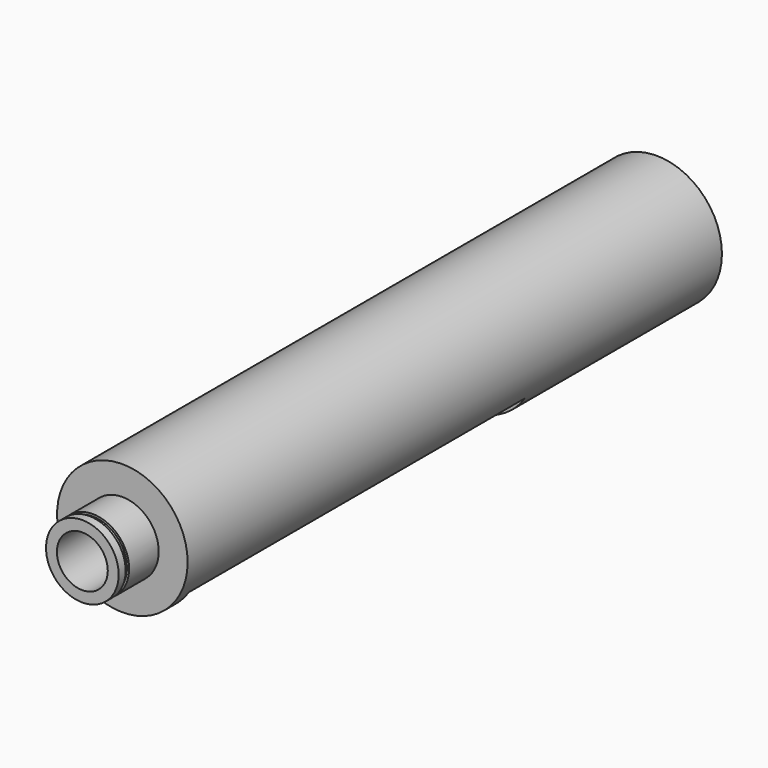
from build123d import *

# Parameters (mm, degrees)
F0_R      = 8.35
F0_R_2    = 5.85
F1_DEPTH  = 15
F2_START  = -11.5
F0_R_3    = 15
F0_R_4    = 12.5
F2_DEPTH  = 3.5
F3_START  = -15
F3_DEPTH  = 150
F4_R      = 15
F4_R_2    = 12.5
F5_DEPTH  = 5
F7_START  = -5
F7_DEPTH  = 51
F8_DEPTH  = 61
F6_W      = 2.95
F6_H      = 4.6
F9_DEPTH  = 15.5
F12_DEPTH = 25
F14_DEPTH = 18.0629715323
F15_DEPTH = 3
F17_START = -2
F16_R     = 8.35
F16_R_2   = 7.85
F17_DEPTH = 1


with BuildPart() as f1:
    # F0 (on Front) → F1 (new body)
    with BuildSketch(Plane.XZ):
        with Locations((-30.6610018015, 20.1133023947)):
            Circle(F0_R)
        with Locations((-30.6610018015, 20.1133023947)):
            Circle(F0_R_2, mode=Mode.SUBTRACT)
    extrude(amount=-F1_DEPTH)

    # F0 (on Front) → F2 (join)
    with BuildSketch(Plane.XZ.offset(F2_START)):
        with Locations((-30.6610018015, 20.1133023947)):
            Circle(F0_R_3)
        with Locations((-30.6610018015, 20.1133023947)):
            Circle(F0_R_4, mode=Mode.SUBTRACT)
        with Locations((-30.6610018015, 20.1133023947)):
            Circle(F0_R_4)
        with Locations((-30.6610018015, 20.1133023947)):
            Circle(F0_R, mode=Mode.SUBTRACT)
    extrude(amount=-F2_DEPTH)

    # F0 (on Front) → F3 (join)
    with BuildSketch(Plane.XZ.offset(F3_START)):
        with Locations((-30.6610018015, 20.1133023947)):
            Circle(F0_R_3)
        with Locations((-30.6610018015, 20.1133023947)):
            Circle(F0_R_4, mode=Mode.SUBTRACT)
    extrude(amount=-F3_DEPTH)

    # F4 (on face) → F5 (join)
    with BuildSketch(Plane(origin=(0, 165, 0), x_dir=(-1, 0, 0), z_dir=(0, 1, 0))):
        with Locations((30.6610018015, 20.1133023947)):
            Circle(F4_R)
        with Locations((30.6610018015, 20.1133023947)):
            Circle(F4_R_2, mode=Mode.SUBTRACT)
        with Locations((30.6610018015, 20.1133023947)):
            Circle(F4_R_2)
    extrude(amount=-F5_DEPTH)

    # F6 (on face) → F7 (join)
    with BuildSketch(Plane(origin=(0, 165, 0), x_dir=(-1, 0, 0), z_dir=(0, 1, 0)).offset(F7_START)):
        with BuildLine():
            Line((38.1610018015, 20.1133023947), (40.1610018015, 20.1133023947))
            ThreePointArc((40.1610018015, 20.1133023947), (30.6610018015, 29.6133023947), (21.1610018015, 20.1133023947))
            Line((21.1610018015, 20.1133023947), (23.1610018015, 20.1133023947))
            ThreePointArc((23.1610018015, 20.1133023947), (23.8256071477, 23.1999478111), (25.7016364485, 25.7395529487))
            Line((25.7016364485, 25.7395529487), (25.7016364485, 26.9397236407))
            Line((25.7016364485, 26.9397236407), (27.2110018015, 26.9397236407))
            Line((27.2110018015, 26.9397236407), (27.2110018015, 26.7726942589))
            ThreePointArc((27.2110018015, 26.7726942589), (30.6610018015, 27.6133023947), (34.1110018015, 26.7726942589))
            Line((34.1110018015, 26.7726942589), (34.1110018015, 26.9397236407))
            Line((34.1110018015, 26.9397236407), (35.6203671545, 26.9397236407))
            Line((35.6203671545, 26.9397236407), (35.6203671545, 25.7395529487))
            ThreePointArc((35.6203671545, 25.7395529487), (37.4963964553, 23.1999478111), (38.1610018015, 20.1133023947))
        make_face()
        with BuildLine():
            ThreePointArc((21.1610018015, 20.1133023947), (30.6610018015, 10.6133023947), (40.1610018015, 20.1133023947))
            Line((40.1610018015, 20.1133023947), (38.1610018015, 20.1133023947))
            ThreePointArc((38.1610018015, 20.1133023947), (30.6610018015, 12.6133023947), (23.1610018015, 20.1133023947))
            Line((23.1610018015, 20.1133023947), (21.1610018015, 20.1133023947))
        make_face()
        with BuildLine():
            Line((25.7016364485, 26.9397236407), (25.7016364485, 25.7395529487))
            ThreePointArc((25.7016364485, 25.7395529487), (26.424706055, 26.3023086436), (27.2110018015, 26.7726942589))
            Line((27.2110018015, 26.7726942589), (27.2110018015, 26.9397236407))
            Line((27.2110018015, 26.9397236407), (25.7016364485, 26.9397236407))
        make_face()
        with BuildLine():
            ThreePointArc((34.1110018015, 26.7726942589), (34.897297548, 26.3023086436), (35.6203671545, 25.7395529487))
            Line((35.6203671545, 25.7395529487), (35.6203671545, 26.9397236407))
            Line((35.6203671545, 26.9397236407), (34.1110018015, 26.9397236407))
            Line((34.1110018015, 26.9397236407), (34.1110018015, 26.7726942589))
        make_face()
    extrude(amount=-F7_DEPTH)

    # F6 (on face) → F8 (join)
    with BuildSketch(Plane(origin=(0, 165, 0), x_dir=(-1, 0, 0), z_dir=(0, 1, 0))):
        with BuildLine():
            Line((34.1110018015, 20.1133023947), (38.1610018015, 20.1133023947))
            ThreePointArc((38.1610018015, 20.1133023947), (37.4963964553, 23.1999478111), (35.6203671545, 25.7395529487))
            Line((35.6203671545, 25.7395529487), (35.6203671545, 25.2133023947))
            Line((35.6203671545, 25.2133023947), (34.1110018015, 25.2133023947))
            Line((34.1110018015, 25.2133023947), (34.1110018015, 20.1133023947))
        make_face()
        with BuildLine():
            Line((35.6203671545, 25.2133023947), (35.6203671545, 25.7395529487))
            ThreePointArc((35.6203671545, 25.7395529487), (34.897297548, 26.3023086436), (34.1110018015, 26.7726942589))
            Line((34.1110018015, 26.7726942589), (34.1110018015, 25.2133023947))
            Line((34.1110018015, 25.2133023947), (35.6203671545, 25.2133023947))
        make_face()
        with BuildLine():
            Line((34.1110018015, 25.2133023947), (34.1110018015, 26.7726942589))
            ThreePointArc((34.1110018015, 26.7726942589), (30.6610018015, 27.6133023947), (27.2110018015, 26.7726942589))
            Line((27.2110018015, 26.7726942589), (27.2110018015, 25.2133023947))
            Line((27.2110018015, 25.2133023947), (30.6610018015, 25.2133023947))
            Line((30.6610018015, 25.2133023947), (34.1110018015, 25.2133023947))
        make_face()
        with BuildLine():
            ThreePointArc((27.2110018015, 26.7726942589), (26.424706055, 26.3023086436), (25.7016364485, 25.7395529487))
            Line((25.7016364485, 25.7395529487), (25.7016364485, 25.2133023947))
            Line((25.7016364485, 25.2133023947), (27.2110018015, 25.2133023947))
            Line((27.2110018015, 25.2133023947), (27.2110018015, 26.7726942589))
        make_face()
        with BuildLine():
            ThreePointArc((25.7016364485, 25.7395529487), (23.8256071477, 23.1999478111), (23.1610018015, 20.1133023947))
            Line((23.1610018015, 20.1133023947), (27.2110018015, 20.1133023947))
            Line((27.2110018015, 20.1133023947), (27.2110018015, 25.2133023947))
            Line((27.2110018015, 25.2133023947), (25.7016364485, 25.2133023947))
            Line((25.7016364485, 25.2133023947), (25.7016364485, 25.7395529487))
        make_face()
        with BuildLine():
            ThreePointArc((23.1610018015, 20.1133023947), (30.6610018015, 12.6133023947), (38.1610018015, 20.1133023947))
            Line((38.1610018015, 20.1133023947), (34.1110018015, 20.1133023947))
            Line((34.1110018015, 20.1133023947), (34.1110018015, 15.0133023947))
            Line((34.1110018015, 15.0133023947), (30.6610018015, 15.0133023947))
            Line((30.6610018015, 15.0133023947), (27.2110018015, 15.0133023947))
            Line((27.2110018015, 15.0133023947), (27.2110018015, 20.1133023947))
            Line((27.2110018015, 20.1133023947), (23.1610018015, 20.1133023947))
        make_face()
    extrude(amount=-F8_DEPTH)

    # F6 (on face) → F9 (cut)
    with BuildSketch(Plane(origin=(0, 165, 0), x_dir=(-1, 0, 0), z_dir=(0, 1, 0))):
        with Locations((32.1360018015, 22.4133023947)):
            Rectangle(F6_W, F6_H)
        Polygon((33.6110018015, 20.1133023947), (34.1110018015, 20.1133023947), (34.1110018015, 25.2133023947), (30.6610018015, 25.2133023947), (27.2110018015, 25.2133023947), (27.2110018015, 20.1133023947), (27.7110018015, 20.1133023947), (27.7110018015, 24.7133023947), (30.6610018015, 24.7133023947), (33.6110018015, 24.7133023947), align=None)
        Polygon((33.6110018015, 15.5133023947), (33.6110018015, 20.1133023947), (30.6610018015, 20.1133023947), (27.7110018015, 20.1133023947), (27.7110018015, 15.5133023947), (30.6610018015, 15.5133023947), align=None)
        with Locations((29.1860018015, 22.4133023947)):
            Rectangle(F6_W, F6_H)
        Polygon((34.1110018015, 15.0133023947), (34.1110018015, 20.1133023947), (33.6110018015, 20.1133023947), (33.6110018015, 15.5133023947), (30.6610018015, 15.5133023947), (27.7110018015, 15.5133023947), (27.7110018015, 20.1133023947), (27.2110018015, 20.1133023947), (27.2110018015, 15.0133023947), (30.6610018015, 15.0133023947), align=None)
    extrude(amount=-F9_DEPTH, mode=Mode.SUBTRACT)

    # F11 (on face) → F12 (cut)
    with BuildSketch(Plane.XY.offset(20.1133023947)):
        Polygon((-43.1610018015, 15), (-18.1610018015, 15), (-18.1610018015, 111.4961504936), (-21.1610018015, 111.4961504936), (-21.1610018015, 93.4331789613), (-40.1610018015, 93.4331789613), (-40.1610018015, 111.4961504936), (-43.1610018015, 111.4961504936), align=None)
    extrude(amount=-F12_DEPTH, mode=Mode.SUBTRACT)

    # F13 (on face) → F14 (cut, through all)
    with BuildSketch(Plane.XZ.offset(-93.4331789613)):
        with BuildLine():
            Line((-40.1610018015, 11.9892639901), (-40.1610018015, 8.5051156285))
            ThreePointArc((-40.1610018015, 8.5051156285), (-30.6610018015, 5.1133023947), (-21.1610018015, 8.5051156285))
            Line((-21.1610018015, 8.5051156285), (-21.1610018015, 11.9892639901))
            ThreePointArc((-21.1610018015, 11.9892639901), (-30.6610018015, 7.6133023947), (-40.1610018015, 11.9892639901))
        make_face()
    extrude(amount=-F14_DEPTH, mode=Mode.SUBTRACT)

    # F6 (on face) → F15 (join)
    with BuildSketch(Plane(origin=(0, 165, 0), x_dir=(-1, 0, 0), z_dir=(0, 1, 0))):
        with BuildLine():
            ThreePointArc((27.2110018015, 26.7726942589), (26.424706055, 26.3023086436), (25.7016364485, 25.7395529487))
            Line((25.7016364485, 25.7395529487), (25.7016364485, 25.2133023947))
            Line((25.7016364485, 25.2133023947), (27.2110018015, 25.2133023947))
            Line((27.2110018015, 25.2133023947), (27.2110018015, 26.7726942589))
        make_face()
        with BuildLine():
            Line((25.7016364485, 26.9397236407), (25.7016364485, 25.7395529487))
            ThreePointArc((25.7016364485, 25.7395529487), (26.424706055, 26.3023086436), (27.2110018015, 26.7726942589))
            Line((27.2110018015, 26.7726942589), (27.2110018015, 26.9397236407))
            Line((27.2110018015, 26.9397236407), (25.7016364485, 26.9397236407))
        make_face()
        with BuildLine():
            Line((35.6203671545, 25.2133023947), (35.6203671545, 25.7395529487))
            ThreePointArc((35.6203671545, 25.7395529487), (34.897297548, 26.3023086436), (34.1110018015, 26.7726942589))
            Line((34.1110018015, 26.7726942589), (34.1110018015, 25.2133023947))
            Line((34.1110018015, 25.2133023947), (35.6203671545, 25.2133023947))
        make_face()
        with BuildLine():
            ThreePointArc((34.1110018015, 26.7726942589), (34.897297548, 26.3023086436), (35.6203671545, 25.7395529487))
            Line((35.6203671545, 25.7395529487), (35.6203671545, 26.9397236407))
            Line((35.6203671545, 26.9397236407), (34.1110018015, 26.9397236407))
            Line((34.1110018015, 26.9397236407), (34.1110018015, 26.7726942589))
        make_face()
    extrude(amount=F15_DEPTH)

    # F16 (on face) → F17 (cut)
    with BuildSketch(Plane.XZ.offset(F17_START)):
        with Locations((-30.6610018015, 20.1133023947)):
            Circle(F16_R)
        with Locations((-30.6610018015, 20.1133023947)):
            Circle(F16_R_2, mode=Mode.SUBTRACT)
    extrude(amount=-F17_DEPTH, mode=Mode.SUBTRACT)


solid = f1.part
